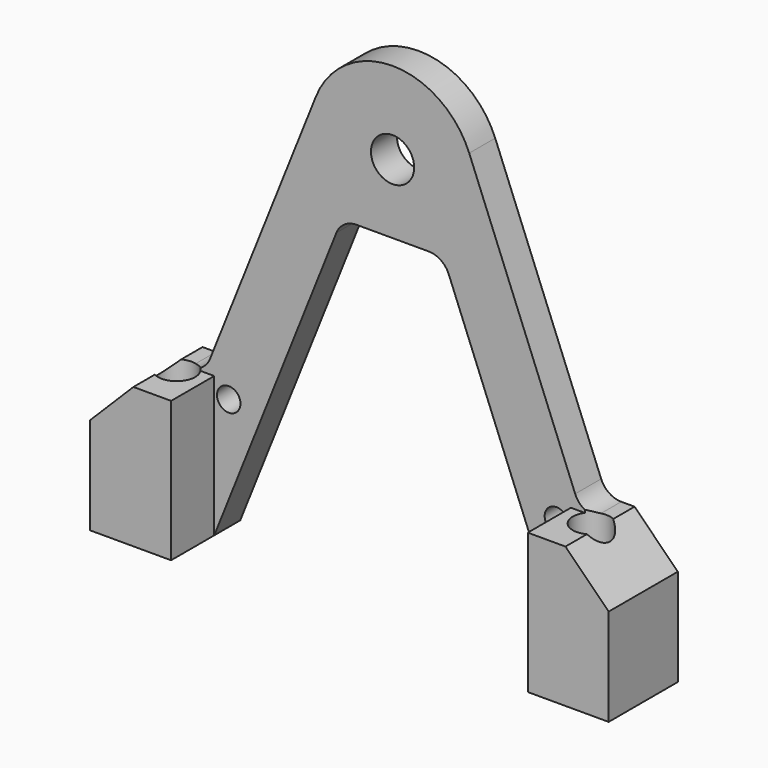
from build123d import *

# Parameters (mm, degrees)
F0_R           = 3.175
F1_DEPTH       = 4.7752
F3_DEPTH       = 7.9248
F4_SIZE        = 6.35
F6_D           = 3.4544
F6_START       = 1.4605
F6_CBORE_D     = 5.461
F6_CBORE_DEPTH = 11.0998
F8_D           = 3.4544
F8_DEPTH       = 5.08
F8_TIP         = 1.0378064612
F9_T4_DEPTH    = 4.7752
F9_S5_R        = 2.7305
F9_T6_DEPTH    = 4
F9_T10_DEPTH   = 4.7752
F9_S11_R       = 2.7305
F9_T12_DEPTH   = 4


# Not quite as in the source:
# - a fillet or chamfer that OpenCascade refuses, or shapes differently, is made with other operations: its cross-section is extruded or revolved along the edge and cut away or added


with BuildPart() as f1:
    # F0 (on Front) → F1 (new body)
    with BuildSketch(Plane.XZ):
        with BuildLine():
            ThreePointArc((-8.2574477487, 44.9918270709), (-7.0896388893, 46.4434074028), (-5.3086, 46.99))
            Line((-5.3086, 46.99), (5.3086, 46.99))
            ThreePointArc((5.3086, 46.99), (7.0896388893, 46.4434074028), (8.2574477487, 44.9918270709))
            Line((8.2574477487, 44.9918270709), (26.2128, 0))
            Line((26.2128, 0), (38.1, 0))
            Line((38.1, 0), (38.1, 20.6248))
            Line((38.1, 20.6248), (27.6356818802, 20.6248))
            Line((27.6356818802, 20.6248), (11.2650625427, 61.6456646408))
            ThreePointArc((11.2650625427, 61.6456646408), (0, 69.2789997383), (-11.2650625427, 61.6456646408))
            Line((-11.2650625427, 61.6456646408), (-27.6356818802, 20.6248))
            Line((-27.6356818802, 20.6248), (-38.1, 20.6248))
            Line((-38.1, 20.6248), (-38.1, 0))
            Line((-38.1, 0), (-26.2128, 0))
            Line((-26.2128, 0), (-8.2574477487, 44.9918270709))
        make_face()
        with Locations((0, 57.15)):
            Circle(F0_R, mode=Mode.SUBTRACT)
    extrude(amount=F1_DEPTH)

    # F2 (on face) → F3 (join)
    with BuildSketch(Plane.XZ.offset(4.7752)):
        Polygon((-27.6356818802, 20.6248), (-38.1, 20.6248), (-38.1, 0), (-26.2128, 0), (-26.2128, 20.6248), align=None)
        Polygon((38.1, 20.6248), (27.6356818802, 20.6248), (26.2128, 20.6248), (26.2128, 0), (38.1, 0), align=None)
    extrude(amount=F3_DEPTH)

    # F4
    f4_edges = [f1.edges().sort_by_distance(p)[0] for p in [
        (38.1, -6.35, 20.6248),
        (-38.1, -6.35, 20.6248),
    ]]
    chamfer(f4_edges, length=F4_SIZE)

    # F6 (through all)
    # its depths count from where the whole tool has entered the part; down to there all is cleared
    with Locations(Plane.XY.offset(20.6248).offset(-F6_START)):
        with Locations((-30.48, -6.35), (30.48, -6.35)):
            CounterBoreHole(F6_D / 2, F6_CBORE_D / 2, F6_CBORE_DEPTH)

    # F8
    with Locations(Plane(origin=(0, 0, 0), x_dir=(-1, 0, 0), z_dir=(0, 1, 0))):
        with Locations((-24.0792, 18.288), (24.0792, 18.288)):
            Hole(F8_D / 2, depth=F8_DEPTH)
            with Locations((0, 0, -(F8_DEPTH + F8_TIP / 2))):  # 118° drill point
                Cone(0, F8_D / 2, F8_TIP, mode=Mode.SUBTRACT)

    # F9: fillet of radius 3.175 on 2 edges, made by hand


with BuildPart() as f9_tool2:
    # F9_s3 → F9_t4 (new body)
    with BuildSketch(Plane.XZ):
        with BuildLine():
            ThreePointArc((-29.7870981589, 20.6248), (-28.0060592696, 21.1713925972), (-26.8382504101, 22.6229729291))
            Line((-26.8382504101, 22.6229729291), (-27.6356818802, 20.6248))
            Line((-27.6356818802, 20.6248), (-29.7870981589, 20.6248))
        make_face()
    extrude(amount=F9_T4_DEPTH)

    # F9_s5 → F9_t6 (cut, symmetric)
    with BuildSketch(Plane.XY.offset(21.6)):
        with Locations((-30.48, -6.35)):
            Circle(F9_S5_R)
    extrude(amount=F9_T6_DEPTH, both=True, mode=Mode.SUBTRACT)


with BuildPart() as f1_1:
    add(f1.part)

    # F9_t1: union F9_tool2
    add(f9_tool2.part)


with BuildPart() as f9_tool8:
    # F9_s9 → F9_t10 (new body)
    with BuildSketch(Plane.XZ):
        with BuildLine():
            ThreePointArc((26.8382504101, 22.6229729291), (28.0060592696, 21.1713925972), (29.7870981589, 20.6248))
            Line((29.7870981589, 20.6248), (27.6356818802, 20.6248))
            Line((27.6356818802, 20.6248), (26.8382504101, 22.6229729291))
        make_face()
    extrude(amount=F9_T10_DEPTH)

    # F9_s11 → F9_t12 (cut, symmetric)
    with BuildSketch(Plane.XY.offset(21.6)):
        with Locations((30.48, -6.35)):
            Circle(F9_S11_R)
    extrude(amount=F9_T12_DEPTH, both=True, mode=Mode.SUBTRACT)


with BuildPart() as f1_2:
    add(f1_1.part)

    # F9_t7: union F9_tool8
    add(f9_tool8.part)


solid = f1_2.part
